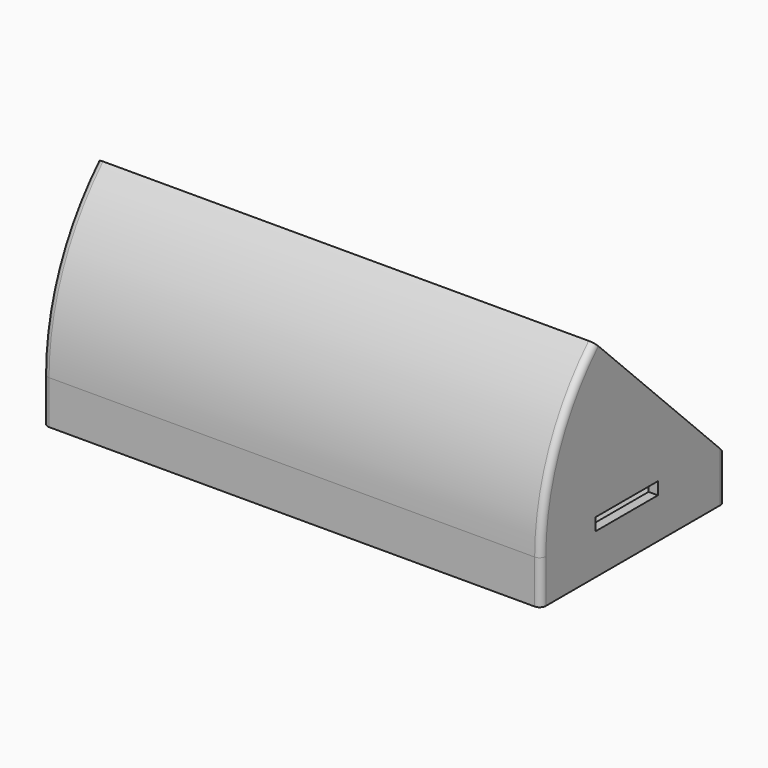
from build123d import *

# Parameters (mm, degrees)
F0_W        = 160
F0_H        = 74
F1_DEPTH    = 2
F2_W        = 97.5
F2_H        = 40
F2_R        = 4.5
F2_R_2      = 3.5
F3_DEPTH    = 2
F4_W        = 9
F4_H        = 9
F5_DEPTH    = 10
F6_R        = 1.75
F7_DEPTH    = 8
F8_W        = 160
F8_H        = 74
F9_DEPTH    = 12
F9_FACE_W   = 160
F9_FACE_H   = 74
F9_FACE_W_2 = 154
F9_FACE_H_2 = 68
F10_ANGLE   = 45
F11_W       = 25
F11_H       = 4
F12_DEPTH   = 3
F13_R       = 2
F14_R       = 4


# Not quite as in the source:
# - a feature names something its author has since deleted; it is built from what else it names


with BuildPart() as f1:
    # F0 (on Top) → F1 (new body)
    with BuildSketch(Plane.XY):
        Rectangle(F0_W, F0_H)
    extrude(amount=F1_DEPTH)

    # F2 (on face) → F3 (cut)
    with BuildSketch(Plane.XY.offset(2)):
        with Locations((12.25, -2)):
            Rectangle(F2_W, F2_H)
        with Locations((-62.5, 2)):
            Circle(F2_R)
        with Locations((-62.5, -15)):
            Circle(F2_R_2)
    extrude(amount=-F3_DEPTH, mode=Mode.SUBTRACT)

    # F4 (on face) → F5 (join)
    with BuildSketch(Plane.XY.offset(2)):
        with Locations((72.5, 29.5)):
            Rectangle(F4_W, F4_H)
        with Locations((-72.5, 29.5)):
            Rectangle(F4_W, F4_H)
        with Locations((-72.5, -20.5)):
            Rectangle(F4_W, F4_H)
        with Locations((72.5, -20.5)):
            Rectangle(F4_W, F4_H)
    extrude(amount=F5_DEPTH)

    # F6 (on face) → F7 (cut)
    with BuildSketch(Plane.XY.offset(12)):
        with Locations((-72.5096613169, 29.5301117003)):
            Circle(F6_R)
        with Locations((-72.5096613169, -20.5968357623)):
            Circle(F6_R)
        with Locations((72.5096613169, 29.5301117003)):
            Circle(F6_R)
        with Locations((72.5096613169, -20.5968357623)):
            Circle(F6_R)
    extrude(amount=-F7_DEPTH, mode=Mode.SUBTRACT)

    # F8 (on face) → F9 (join)
    with BuildSketch(Plane.XY.offset(2)):
        Rectangle(F8_W, F8_H)
        Polygon((-77, 25), (-77, 34), (-68, 34), (68, 34), (77, 34), (77, 25), (77, -16), (77, -25), (77, -34), (-77, -34), (-77, -25), (-77, -16), align=None, mode=Mode.SUBTRACT)
    extrude(amount=F9_DEPTH)

    # F9_face (on face) → F10 (revolve)
    with BuildSketch(Plane.XY.offset(14)):
        Rectangle(F9_FACE_W, F9_FACE_H)
        Rectangle(F9_FACE_W_2, F9_FACE_H_2, mode=Mode.SUBTRACT)
    revolve(axis=Axis((0, 37, 14), (-1, 0, 0)), revolution_arc=F10_ANGLE)

    # F11 (on face) → F12 (cut)
    with BuildSketch(Plane.YZ.offset(80)):
        with Locations((-2.5, 15)):
            Rectangle(F11_W, F11_H)
    extrude(amount=-F12_DEPTH, mode=Mode.SUBTRACT)

    # F13
    f13_edges = [f1.edges().sort_by_distance(p)[0] for p in [
        (80, 37, 7),
        (80, -31.367085, 42.318574),
        (80, -37, 7),
        (-80, 37, 7),
        (-80, -31.367085, 42.318574),
        (-80, -37, 7),
        (-77, 34.228361, 15.14805),
        (77, 34.228361, 15.14805),
    ]]
    fillet(f13_edges, radius=F13_R)

    # F14
    f14_edges = [f1.edges().sort_by_distance(p)[0] for p in [
        (-77, -28.595447, 41.170524),
        (77, -28.595447, 41.170524),
    ]]
    fillet(f14_edges, radius=F14_R)


solid = f1.part
